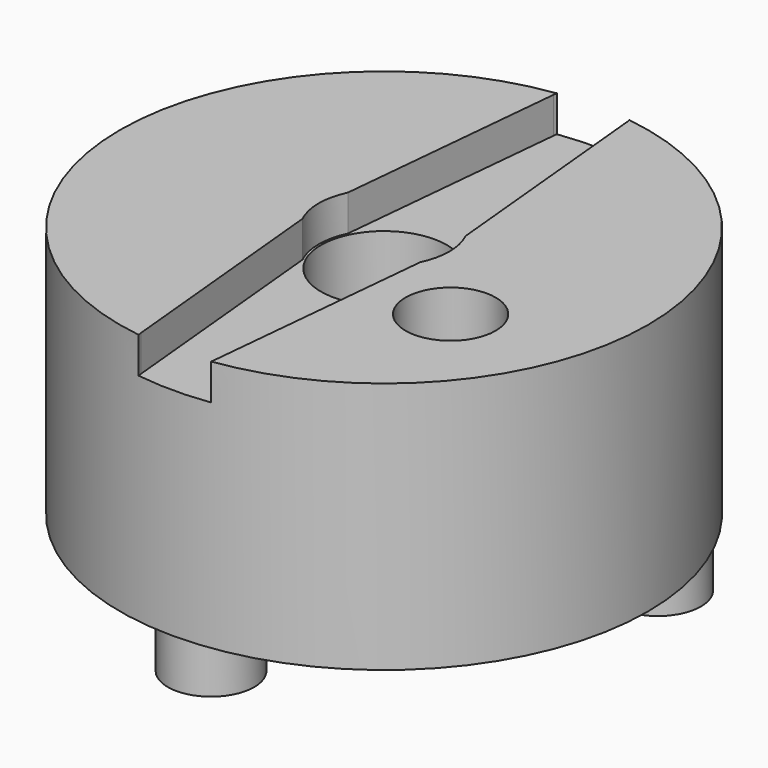
from build123d import *

# Parameters (mm, degrees)
F0_R     = 14.65
F1_DEPTH = 14
F2_R     = 2.4
F2_R_2   = 0.7
F3_DEPTH = 2.8
F4_R     = 3.5
F4_R_2   = 2.5
F5_DEPTH = 25
F7_DEPTH = 2


# Not quite as in the source:
# - a feature of the source that left no trace in its solid (it failed there, or was rolled back) is left out


with BuildPart() as f1:
    # F0 (on Top) → F1 (new body)
    with BuildSketch(Plane.XY):
        Circle(F0_R)
    extrude(amount=F1_DEPTH)

    # F2 (on face) → F3 (join)
    with BuildSketch(Plane(origin=(0, 0, 0), x_dir=(1, 0, 0), z_dir=(0, 0, -1))):
        with Locations((0, 12)):
            Circle(F2_R)
        with Locations((0, 12)):
            Circle(F2_R_2, mode=Mode.SUBTRACT)
        with Locations((-10.3923048454, -6)):
            Circle(F2_R)
        with Locations((-10.3923048454, -6)):
            Circle(F2_R_2, mode=Mode.SUBTRACT)
        with Locations((10.3923048454, -6)):
            Circle(F2_R)
        with Locations((10.3923048454, -6)):
            Circle(F2_R_2, mode=Mode.SUBTRACT)
    extrude(amount=F3_DEPTH)

    # F4 (on face) → F5 (cut)
    with BuildSketch(Plane.XY.offset(14)):
        Circle(F4_R)
        with Locations((7.3377376988, -4.5508025283)):
            Circle(F4_R_2)
    extrude(amount=-F5_DEPTH, mode=Mode.SUBTRACT)

    # F6 (on face) → F7 (cut)
    with BuildSketch(Plane.XY.offset(14)):
        with BuildLine():
            ThreePointArc((3.265158964, -1.5745989775), (3.533894894, -0.8075963582), (3.625, 0))
            ThreePointArc((3.625, 0), (3.533894894, 0.8075963582), (3.265158964, 1.5745989775))
            ThreePointArc((3.265158964, 1.5745989775), (0, 3.625), (-3.265158964, 1.5745989775))
            ThreePointArc((-3.265158964, 1.5745989775), (-3.625, 0), (-3.265158964, -1.5745989775))
            ThreePointArc((-3.265158964, -1.5745989775), (0, -3.625), (3.265158964, -1.5745989775))
        make_face()
        with BuildLine():
            ThreePointArc((-3.265158964, 1.5745989775), (0, 3.625), (3.265158964, 1.5745989775))
            Line((3.265158964, 1.5745989775), (2.0405680426, 14.2964231749))
            ThreePointArc((2.0405680426, 14.2964231749), (2.047640653, 14.1983247495), (2.05, 14.1))
            ThreePointArc((2.05, 14.1), (-0.0983247495, 12.052359347), (-2.0405680426, 14.2964231749))
            Line((-2.0405680426, 14.2964231749), (-3.265158964, 1.5745989775))
        make_face()
        with BuildLine():
            Line((2.0405680426, -14.2964231749), (3.265158964, -1.5745989775))
            ThreePointArc((3.265158964, -1.5745989775), (0, -3.625), (-3.265158964, -1.5745989775))
            Line((-3.265158964, -1.5745989775), (-2.0405680426, -14.2964231749))
            ThreePointArc((-2.0405680426, -14.2964231749), (-0.0983247495, -12.052359347), (2.05, -14.1))
            ThreePointArc((2.05, -14.1), (2.047640653, -14.1983247495), (2.0405680426, -14.2964231749))
        make_face()
        with BuildLine():
            ThreePointArc((2.05, 14.1), (2.047640653, 14.1983247495), (2.0405680426, 14.2964231749))
            ThreePointArc((2.0405680426, 14.2964231749), (0, 16.15), (-2.0405680426, 14.2964231749))
            ThreePointArc((-2.0405680426, 14.2964231749), (-0.0983247495, 12.052359347), (2.05, 14.1))
        make_face()
        with BuildLine():
            ThreePointArc((-2.0405680426, -14.2964231749), (0, -16.15), (2.0405680426, -14.2964231749))
            ThreePointArc((2.0405680426, -14.2964231749), (2.047640653, -14.1983247495), (2.05, -14.1))
            ThreePointArc((2.05, -14.1), (-0.0983247495, -12.052359347), (-2.0405680426, -14.2964231749))
        make_face()
    extrude(amount=-F7_DEPTH, mode=Mode.SUBTRACT)


solid = f1.part
